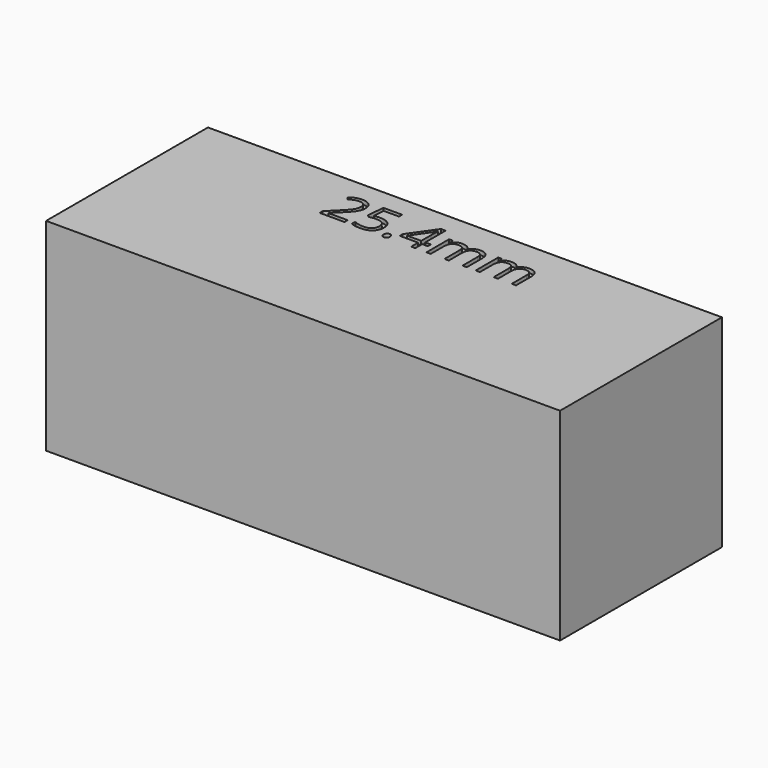
from build123d import *

# Parameters (mm, degrees)
F0_W         = 25.4
F0_H         = 10
F1_DEPTH     = 10
F2_TEXT_SIZE = 2.6141655094
F3_DEPTH     = 0.2


# Not quite as in the source:
# - Text() gives the source's letters only with a copy of the font that has no kerning and outlines rounded to 1/6400 em; it was checked with that copy


with BuildPart() as f1:
    # F0 (on Top) → F1 (new body)
    with BuildSketch(Plane.XY):
        Rectangle(F0_W, F0_H)
    extrude(amount=F1_DEPTH)

    # F2 (on face) → F3 (cut)
    with BuildSketch(Plane.XY.offset(10)):
        with Locations((-5, 2.1178008333)):
            Text('25.4mm', F2_TEXT_SIZE, font='Open Sans', text_align=(TextAlign.LEFT, TextAlign.BOTTOM))
    extrude(amount=-F3_DEPTH, mode=Mode.SUBTRACT)


solid = f1.part
